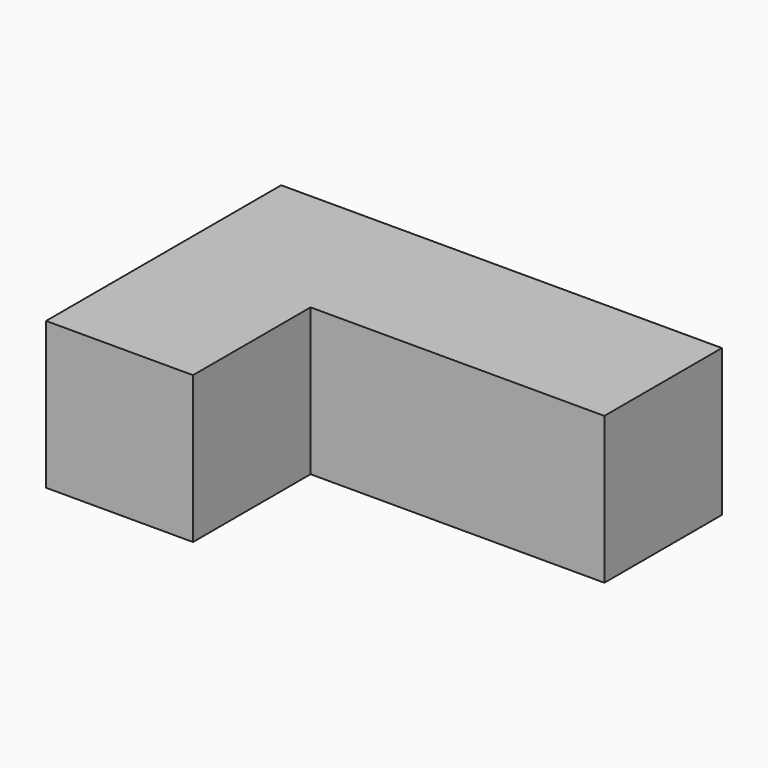
from build123d import *

# Parameters (mm, degrees)
F1_W     = 228.6
F1_H     = 76.2
F2_DEPTH = 76.2
F3_W     = 76.2
F3_H     = 76.2
F4_DEPTH = 76.2


# Not quite as in the source:
# - a variable given as a bare number and used for a length is read in inches; the dataset says mm whatever the document's units were


with BuildPart() as f2:
    # F1 (on Front) → F2 (new body)
    with BuildSketch(Plane.XZ):
        Rectangle(F1_W, F1_H)
    extrude(amount=F2_DEPTH)

    # F3 (on face) → F4 (join)
    with BuildSketch(Plane.XZ.offset(76.2)):
        with Locations((-76.2, 0)):
            Rectangle(F3_W, F3_H)
    extrude(amount=F4_DEPTH)


solid = f2.part
